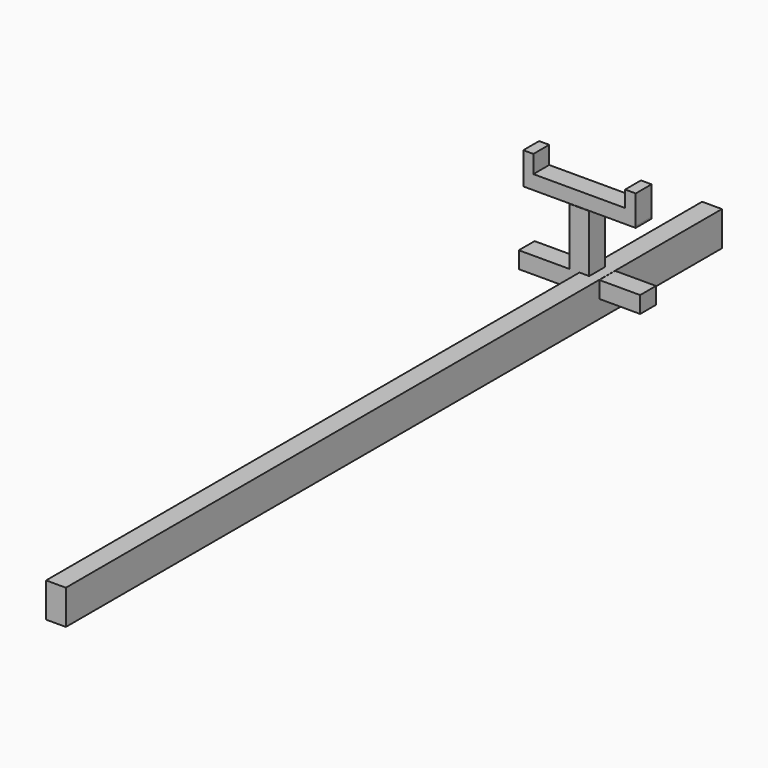
from build123d import *

# Parameters (mm, degrees)
F0_W     = 24.9986350536
F0_H     = 73.6169979911
F0_H_2   = 20.8740851838
F1_DEPTH = 25.4
F0_W_2   = 12.948423624
F0_H_3   = 22.8137746453
F0_H_4   = 1.4562010765
F0_W_3   = 13.506911695
F0_H_5   = 16.0137787461
F2_W     = 1051.9908871502
F2_H     = 44.3331450224
F3_DEPTH = 25.4


# Not quite as in the source:
# - a feature of the source that left no trace in its solid (it failed there, or was rolled back) is left out


with BuildPart() as f1:
    # F0 (on Front) → F1 (new body)
    with BuildSketch(Plane.XZ):
        Polygon((-12.4993175268, -46.8391307633), (-77.8370201588, -46.8391307633), (-77.8370201588, -68.2005307633), (77.8370201588, -68.2005307633), (77.8370201588, -46.8391307633), (12.4993175268, -46.8391307633), (12.4993175268, -67.7132159472), (-12.4993175268, -67.7132159472), align=None)
        with Locations((0, -10.0306317678)):
            Rectangle(F0_W, F0_H)
        with Locations((0, -57.2761733552)):
            Rectangle(F0_W, F0_H_2)
    extrude(amount=F1_DEPTH)

    # F2 (on Right) → F3 (join)
    with BuildSketch(Plane.YZ):
        with Locations((-354.7138301656, -68.8458159566)):
            Rectangle(F2_W, F2_H)
    extrude(amount=F3_DEPTH)


with BuildPart() as f1b:
    # F0 (on Front) → F1, piece 2 (new body)
    with BuildSketch(Plane.XZ):
        with Locations((-65.5878484249, 56.6299296916)):
            Rectangle(F0_W_2, F0_H_3)
        with Locations((-65.5878484249, 44.4949418306)):
            Rectangle(F0_W_2, F0_H_4)
        Polygon((58.5551485419, 45.2230423689), (-59.1136366129, 45.2230423689), (-59.1136366129, 43.7668412924), (-72.0620602369, 43.7668412924), (-72.0620602369, 27.1014645696), (72.0620602369, 27.1014645696), (72.0620602369, 29.2092636228), (58.5551485419, 29.2092636228), align=None)
        Polygon((58.5551485419, 66.097907722), (58.5551485419, 45.2230423689), (72.0620602369, 45.2230423689), (72.0620602369, 29.2092636228), (72.1509829164, 29.2092636228), (72.1509829164, 66.097907722), align=None)
        with Locations((65.3086043894, 37.2161529958)):
            Rectangle(F0_W_3, F0_H_5)
    extrude(amount=F1_DEPTH)


solid = Compound([f1.part, f1b.part])
